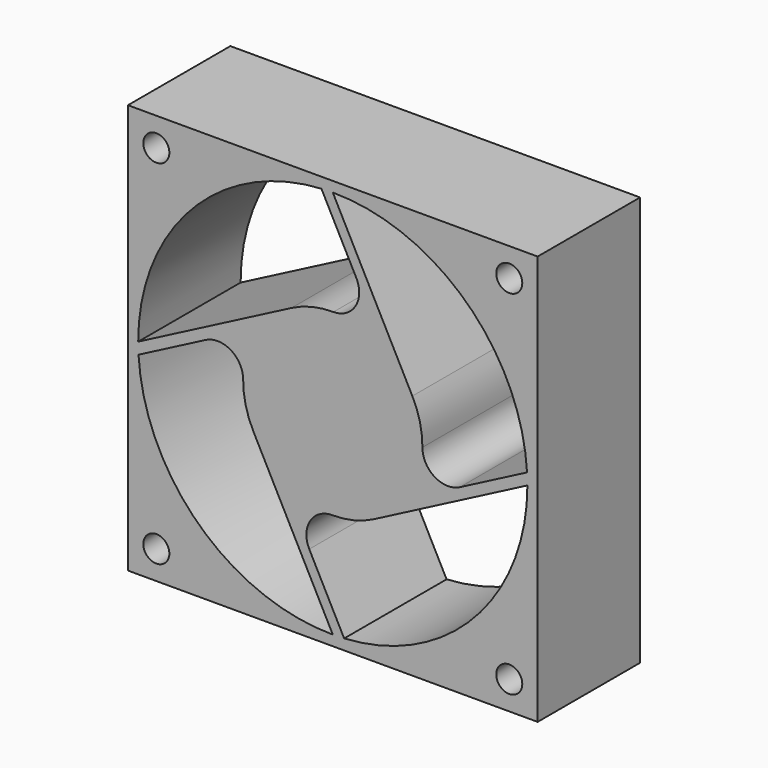
from build123d import *

# Parameters (mm, degrees)
F0_W     = 80
F0_H     = 80
F0_R     = 2.5423391552
F1_DEPTH = 12.5
F2_R     = 5


with BuildPart() as f1:
    # F0 (on Front) → F1 (new body, symmetric)
    with BuildSketch(Plane.XZ):
        Rectangle(F0_W, F0_H)
        with Locations((-34.4576608448, -34.4576608448)):
            Circle(F0_R, mode=Mode.SUBTRACT)
        with BuildLine():
            Line((-37.9351268711, -2.219493022), (-14.3494285056, 10.01718032))
            ThreePointArc((-14.3494285056, 10.01718032), (-17.4625571186, 1.1441585906), (-15.5338058985, -8.0592105263))
            Line((-15.5338058985, -8.0592105263), (0, -38))
            ThreePointArc((0, -38), (-26.0735427701, -27.6436315888), (-37.9351268711, -2.219493022))
        make_face(mode=Mode.SUBTRACT)
        with Locations((34.4576608448, -34.4576608448)):
            Circle(F0_R, mode=Mode.SUBTRACT)
        with BuildLine():
            Line((8.0592105263, -15.5338058985), (38, 0))
            ThreePointArc((38, 0), (27.6436315888, -26.0735427701), (2.219493022, -37.9351268711))
            Line((2.219493022, -37.9351268711), (-10.01718032, -14.3494285056))
            ThreePointArc((-10.01718032, -14.3494285056), (-1.1441585906, -17.4625571186), (8.0592105263, -15.5338058985))
        make_face(mode=Mode.SUBTRACT)
        with BuildLine():
            Line((-8.0592105263, 15.5338058985), (-38, 0))
            ThreePointArc((-38, 0), (-27.6436315888, 26.0735427701), (-2.219493022, 37.9351268711))
            Line((-2.219493022, 37.9351268711), (10.01718032, 14.3494285056))
            ThreePointArc((10.01718032, 14.3494285056), (1.1441585906, 17.4625571186), (-8.0592105263, 15.5338058985))
        make_face(mode=Mode.SUBTRACT)
        with Locations((-34.4576608448, 34.4576608448)):
            Circle(F0_R, mode=Mode.SUBTRACT)
        with BuildLine():
            Line((15.5338058985, 8.0592105263), (0, 38))
            ThreePointArc((0, 38), (26.0735427701, 27.6436315888), (37.9351268711, 2.219493022))
            Line((37.9351268711, 2.219493022), (14.3494285056, -10.01718032))
            ThreePointArc((14.3494285056, -10.01718032), (17.4625571186, -1.1441585906), (15.5338058985, 8.0592105263))
        make_face(mode=Mode.SUBTRACT)
        with Locations((34.4576608448, 34.4576608448)):
            Circle(F0_R, mode=Mode.SUBTRACT)
    extrude(amount=F1_DEPTH, both=True)

    # F2
    f2_edges = [f1.edges().sort_by_distance(p)[0] for p in [
        (10.01718, 0, 14.349429),
        (-14.349429, 0, 10.01718),
        (-10.01718, 0, -14.349429),
        (14.349429, 0, -10.01718),
    ]]
    fillet(f2_edges, radius=F2_R)


solid = f1.part
